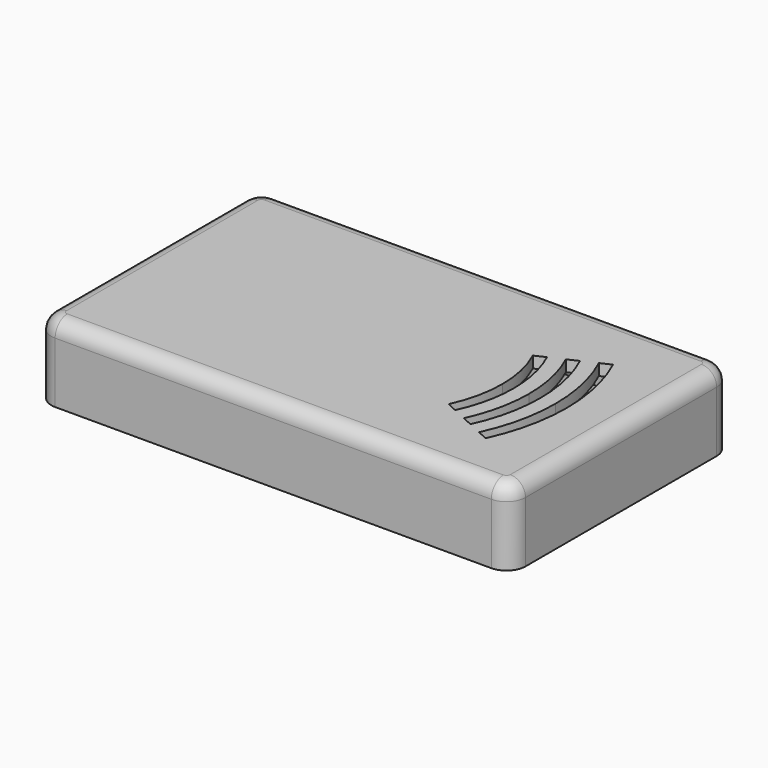
from build123d import *

# Parameters (mm, degrees)
F0_W         = 62.5
F0_H         = 36.5
F0_W_2       = 58.5
F0_H_2       = 31.5
F1_DEPTH     = 7
F3_DEPTH     = 1.5
F4_W         = 62.5
F4_H         = 36.5
F5_DEPTH     = 3
F7_DEPTH     = 2.5
F8_R         = 2.5
F9_T1_DEPTH  = 57.5
F9_T3_DEPTH  = 31.5
F9_T6_ANGLE  = 90
F9_T8_ANGLE  = 90
F9_T10_ANGLE = 90
F9_T12_ANGLE = 90
F10_W        = 1.25
F10_H        = 8.5
F11_DEPTH    = 2
F13_DEPTH    = 3


# Not quite as in the source:
# - a fillet or chamfer that OpenCascade refuses, or shapes differently, is made with other operations: its cross-section is extruded or revolved along the edge and cut away or added
# - a feature names something its author has since deleted; it is built from what else it names


with BuildPart() as f1:
    # F0 (on Top) → F1 (new body)
    with BuildSketch(Plane.XY):
        with Locations((0.5, 0.5)):
            Rectangle(F0_W, F0_H)
        with Locations((1, 0.5)):
            Rectangle(F0_W_2, F0_H_2, mode=Mode.SUBTRACT)
    extrude(amount=F1_DEPTH)

    # F2 (on face) → F3 (join)
    with BuildSketch(Plane.XY.offset(7)):
        Polygon((30.25, 16.25), (-28.25, 16.25), (-28.25, -15.25), (30.25, -15.25), (30.25, -6), (30.25, 7), align=None)
    extrude(amount=-F3_DEPTH)

    # F4 (on face) → F5 (join)
    with BuildSketch(Plane(origin=(0, 0, 0), x_dir=(1, 0, 0), z_dir=(0, 0, -1))):
        with Locations((0.5, -0.5)):
            Rectangle(F4_W, F4_H)
        Polygon((-29.5, -17.522141248), (-29.5, 16.5), (30.25, 16.5), (30.25, 15.25), (30.25, -16.25), (30.25, -17.522141248), align=None, mode=Mode.SUBTRACT)
    extrude(amount=F5_DEPTH)

    # F6 (on face) → F7 (cut)
    with BuildSketch(Plane.YZ.offset(-28.25)):
        with BuildLine():
            Line((4, 5.5), (-3, 5.5))
            ThreePointArc((-3, 5.5), (-3.5303300859, 5.2803300859), (-3.75, 4.75))
            Line((-3.75, 4.75), (-3.75, 3.5))
            ThreePointArc((-3.75, 3.5), (-3.1642135624, 2.0857864376), (-1.75, 1.5))
            Line((-1.75, 1.5), (2.75, 1.5))
            ThreePointArc((2.75, 1.5), (4.1642135624, 2.0857864376), (4.75, 3.5))
            Line((4.75, 3.5), (4.75, 4.75))
            ThreePointArc((4.75, 4.75), (4.5303300859, 5.2803300859), (4, 5.5))
        make_face()
    extrude(amount=-F7_DEPTH, mode=Mode.SUBTRACT)

    # F8
    f8_edges = [f1.edges().sort_by_distance(p)[0] for p in [
        (-30.75, 18.75, 2),
        (-30.75, -17.75, 2),
        (31.75, 18.75, 2),
        (31.75, -17.75, 2),
    ]]
    fillet(f8_edges, radius=F8_R)

    # F9: fillet of radius 2 on 8 edges, made by hand

    # F9_s2 → F9_t1 (cut)
    with BuildSketch(Plane.YZ.offset(-28.25)):
        with BuildLine():
            ThreePointArc((18.75, 5), (18.1642135624, 6.4142135624), (16.75, 7))
            Line((16.75, 7), (18.75, 7))
            Line((18.75, 7), (18.75, 5))
        make_face()
        with BuildLine():
            ThreePointArc((-15.75, 7), (-17.1642135624, 6.4142135624), (-17.75, 5))
            Line((-17.75, 5), (-17.75, 7))
            Line((-17.75, 7), (-15.75, 7))
        make_face()
    extrude(amount=F9_T1_DEPTH, mode=Mode.SUBTRACT)

    # F9_s4 → F9_t3 (cut)
    with BuildSketch(Plane.XZ.offset(-16.25)):
        with BuildLine():
            ThreePointArc((29.75, 7), (31.1642135624, 6.4142135624), (31.75, 5))
            Line((31.75, 5), (31.75, 7))
            Line((31.75, 7), (29.75, 7))
        make_face()
        with BuildLine():
            ThreePointArc((-28.75, 7), (-30.1642135624, 6.4142135624), (-30.75, 5))
            Line((-30.75, 5), (-30.75, 7))
            Line((-30.75, 7), (-28.75, 7))
        make_face()
    extrude(amount=F9_T3_DEPTH, mode=Mode.SUBTRACT)

    # F9_s5 → F9_t6 (revolve, cut)
    with BuildSketch(Plane.YZ.offset(29.25)):
        with BuildLine():
            ThreePointArc((16.75, 7), (18.1642135624, 6.4142135624), (18.75, 5))
            Line((18.75, 5), (18.75, 7))
            Line((18.75, 7), (16.75, 7))
        make_face()
    revolve(axis=Axis((29.25, 16.25, 7), (0, 0, -1)), revolution_arc=F9_T6_ANGLE, mode=Mode.SUBTRACT)

    # F9_s7 → F9_t8 (revolve, cut)
    with BuildSketch(Plane.YZ.offset(-28.25)):
        with BuildLine():
            ThreePointArc((16.75, 7), (18.1642135624, 6.4142135624), (18.75, 5))
            Line((18.75, 5), (18.75, 7))
            Line((18.75, 7), (16.75, 7))
        make_face()
    revolve(axis=Axis((-28.25, 16.25, 7), (0, 0, 1)), revolution_arc=F9_T8_ANGLE, mode=Mode.SUBTRACT)

    # F9_s9 → F9_t10 (revolve, cut)
    with BuildSketch(Plane.XZ.offset(15.25)):
        with BuildLine():
            ThreePointArc((29.75, 7), (31.1642135624, 6.4142135624), (31.75, 5))
            Line((31.75, 5), (31.75, 7))
            Line((31.75, 7), (29.75, 7))
        make_face()
    revolve(axis=Axis((29.25, -15.25, 7), (0, 0, -1)), revolution_arc=F9_T10_ANGLE, mode=Mode.SUBTRACT)

    # F9_s11 → F9_t12 (revolve, cut)
    with BuildSketch(Plane.XZ.offset(15.25)):
        with BuildLine():
            ThreePointArc((-28.75, 7), (-30.1642135624, 6.4142135624), (-30.75, 5))
            Line((-30.75, 5), (-30.75, 7))
            Line((-30.75, 7), (-28.75, 7))
        make_face()
    revolve(axis=Axis((-28.25, -15.25, 7), (0, 0, 1)), revolution_arc=F9_T12_ANGLE, mode=Mode.SUBTRACT)

    # F10 (on face) → F11 (cut)
    with BuildSketch(Plane(origin=(0, 0, 0), x_dir=(1, 0, 0), z_dir=(0, 0, -1))):
        with Locations((-28.875, -0.5)):
            Rectangle(F10_W, F10_H)
    extrude(amount=-F11_DEPTH, mode=Mode.SUBTRACT)

    # F12 (on face) → F13 (cut)
    with BuildSketch(Plane.XY.offset(7)):
        with BuildLine():
            ThreePointArc((22.6871086181, -10.5021475209), (24.4149310408, -5.3769082449), (25, 0))
            ThreePointArc((25, 0), (24.4149310408, 5.3769082449), (22.6871086181, 10.5021475209))
            Line((22.6871086181, 10.5021475209), (21.325882101, 9.8720186697))
            ThreePointArc((21.325882101, 9.8720186697), (22.9500351783, 5.0542937502), (23.5, 0))
            ThreePointArc((23.5, 0), (22.9500351783, -5.0542937502), (21.325882101, -9.8720186697))
            Line((21.325882101, -9.8720186697), (22.6871086181, -10.5021475209))
        make_face()
        with BuildLine():
            ThreePointArc((19.5109134115, -9.031846868), (20.9968406951, -4.6241410906), (21.5, 0))
            ThreePointArc((21.5, 0), (20.9968406951, 4.6241410906), (19.5109134115, 9.031846868))
            Line((19.5109134115, 9.031846868), (18.1496868945, 8.4017180168))
            ThreePointArc((18.1496868945, 8.4017180168), (19.5319448326, 4.3015265959), (20, 0))
            ThreePointArc((20, 0), (19.5319448326, -4.3015265959), (18.1496868945, -8.4017180168))
            Line((18.1496868945, -8.4017180168), (19.5109134115, -9.031846868))
        make_face()
        with BuildLine():
            ThreePointArc((16.334718205, -7.5615462151), (17.5787503494, -3.8713739363), (18, 0))
            ThreePointArc((18, 0), (17.5787503494, 3.8713739363), (16.334718205, 7.5615462151))
            Line((16.334718205, 7.5615462151), (14.9734916879, 6.9314173638))
            ThreePointArc((14.9734916879, 6.9314173638), (16.1138544869, 3.5487594416), (16.5, 0))
            ThreePointArc((16.5, 0), (16.1138544869, -3.5487594416), (14.9734916879, -6.9314173638))
            Line((14.9734916879, -6.9314173638), (16.334718205, -7.5615462151))
        make_face()
    extrude(amount=-F13_DEPTH, mode=Mode.SUBTRACT)


solid = f1.part
